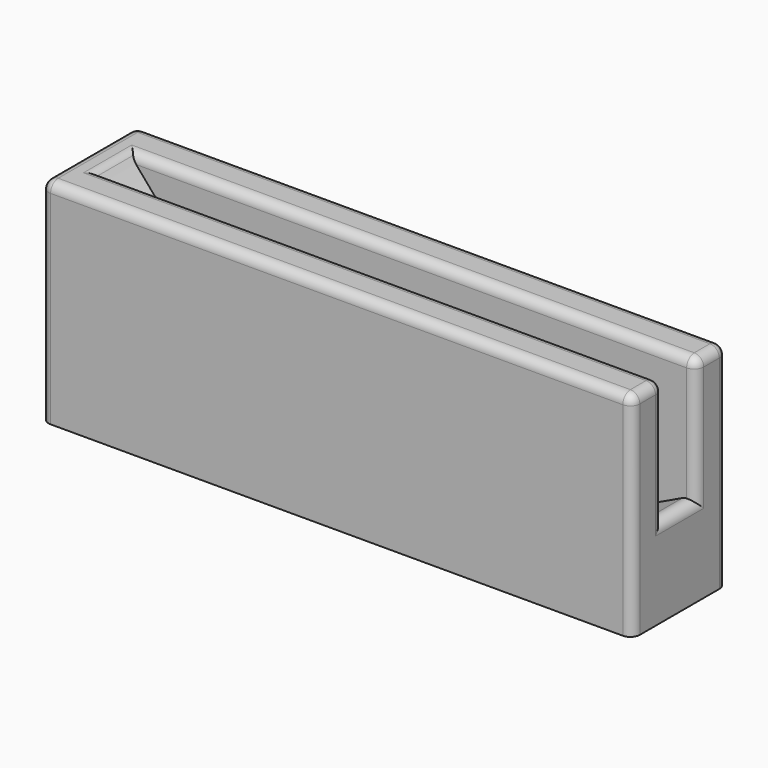
from build123d import *

# Parameters (mm, degrees)
F0_W          = 152.4
F0_H          = 31.75
F1_DEPTH      = 57.15
F3_DEPTH      = 5.55625
F3_DEPTH_BACK = 5.55625
F4_DEPTH      = 6.35
F5_R          = 2.54
F6_T1_DEPTH   = 60.96
F6_S5_W       = 2.54
F6_S5_H       = 2.54
F6_T6_DEPTH   = 2.54
F6_S11_W      = 2.54
F6_S11_H      = 2.54
F6_T12_DEPTH  = 2.54


# Not quite as in the source:
# - a fillet or chamfer that OpenCascade refuses, or shapes differently, is made with other operations: its cross-section is extruded or revolved along the edge and cut away or added


with BuildPart() as f1:
    # F0 (on Top) → F1 (new body)
    with BuildSketch(Plane.XY):
        Rectangle(F0_W, F0_H)
    extrude(amount=F1_DEPTH)

    # F2 (on Front) → F3 (cut, two sides)
    with BuildSketch(Plane.XZ) as f3_sk:
        with BuildLine():
            Line((76.2, 57.2062885404), (0, 57.2062885404))
            Line((0, 57.2062885404), (-76.2, 57.2062885404))
            ThreePointArc((-76.2, 57.2062885404), (-5.9418927192, 12.810203488), (76.2, 25.4562885404))
            Line((76.2, 25.4562885404), (76.2, 57.2062885404))
        make_face()
    extrude(amount=F3_DEPTH, mode=Mode.SUBTRACT)
    extrude(f3_sk.sketch, amount=-F3_DEPTH_BACK, mode=Mode.SUBTRACT)

    # F4 (add): a face of the model
    f4_faces = [f1.faces().sort_by_distance(p)[0] for p in [
        (-76.2, 0, 28.575),
    ]]
    extrude(f4_faces, amount=F4_DEPTH)

    # F5
    f5_edges = [f1.edges().sort_by_distance(p)[0] for p in [
        (76.2, -10.715625, 57.15),
        (-3.175, -15.875, 57.15),
        (76.2, -15.875, 28.575),
        (76.2, 10.715625, 57.15),
        (76.2, 15.875, 28.575),
        (-3.175, 15.875, 57.15),
        (-82.55, 0, 57.15),
        (0.021369, -5.55625, 57.15),
        (-76.157263, 0, 57.15),
        (0.021369, 5.55625, 57.15),
        (76.2, 5.55625, 41.303144),
        (76.2, -5.55625, 41.303144),
        (76.2, 0, 25.456289),
    ]]
    fillet(f5_edges, radius=F5_R)

    # F6: fillet of radius 2.54 on 2 edges, made by hand

    # F6_s2 → F6_t1 (cut)
    with BuildSketch(Plane.XY.offset(-6.35)):
        with BuildLine():
            ThreePointArc((-80.01, 15.875), (-81.8060512242, 15.1310512242), (-82.55, 13.335))
            Line((-82.55, 13.335), (-82.55, 15.875))
            Line((-82.55, 15.875), (-80.01, 15.875))
        make_face()
        with BuildLine():
            ThreePointArc((-82.55, -13.335), (-81.8060512242, -15.1310512242), (-80.01, -15.875))
            Line((-80.01, -15.875), (-82.55, -15.875))
            Line((-82.55, -15.875), (-82.55, -13.335))
        make_face()
    extrude(amount=F6_T1_DEPTH, mode=Mode.SUBTRACT)


with BuildPart() as f6_tool4:
    # F6_s5 → F6_t6 (new body)
    with BuildSketch(Plane.YZ.offset(-80.01)):
        with Locations((-14.605, 55.88)):
            Rectangle(F6_S5_W, F6_S5_H)
    extrude(amount=-F6_T6_DEPTH)

    # F6_s7 → F6_t8 (revolve, cut)
    with BuildSketch(Plane(origin=(-80.01, -13.335, 54.61), x_dir=(0, 0.7071067812, -0.7071067812), z_dir=(0, 0.7071067812, 0.7071067812))):
        with BuildLine():
            ThreePointArc((0, -2.54), (2.54, 0), (0, 2.54))
            Line((0, 2.54), (0, -2.54))
        make_face()
    revolve(axis=Axis((-80.01, -13.335, 54.61), (-1, 0, 0)), mode=Mode.SUBTRACT)


with BuildPart() as f1_1:
    add(f1.part)

    # F6_t3: cut F6_tool4
    add(f6_tool4.part, mode=Mode.SUBTRACT)


with BuildPart() as f6_tool10:
    # F6_s11 → F6_t12 (new body)
    with BuildSketch(Plane.XZ.offset(-13.335)):
        with Locations((-81.28, 55.88)):
            Rectangle(F6_S11_W, F6_S11_H)
    extrude(amount=-F6_T12_DEPTH)

    # F6_s13 → F6_t14 (revolve, cut)
    with BuildSketch(Plane(origin=(-80.01, 13.335, 54.61), x_dir=(0.7071067812, 0, -0.7071067812), z_dir=(0.7071067812, 0, 0.7071067812))):
        with BuildLine():
            ThreePointArc((0, -2.54), (2.54, 0), (0, 2.54))
            Line((0, 2.54), (0, -2.54))
        make_face()
    revolve(axis=Axis((-80.01, 13.335, 54.61), (0, 1, 0)), mode=Mode.SUBTRACT)


with BuildPart() as f1_2:
    add(f1_1.part)

    # F6_t9: cut F6_tool10
    add(f6_tool10.part, mode=Mode.SUBTRACT)


solid = f1_2.part
